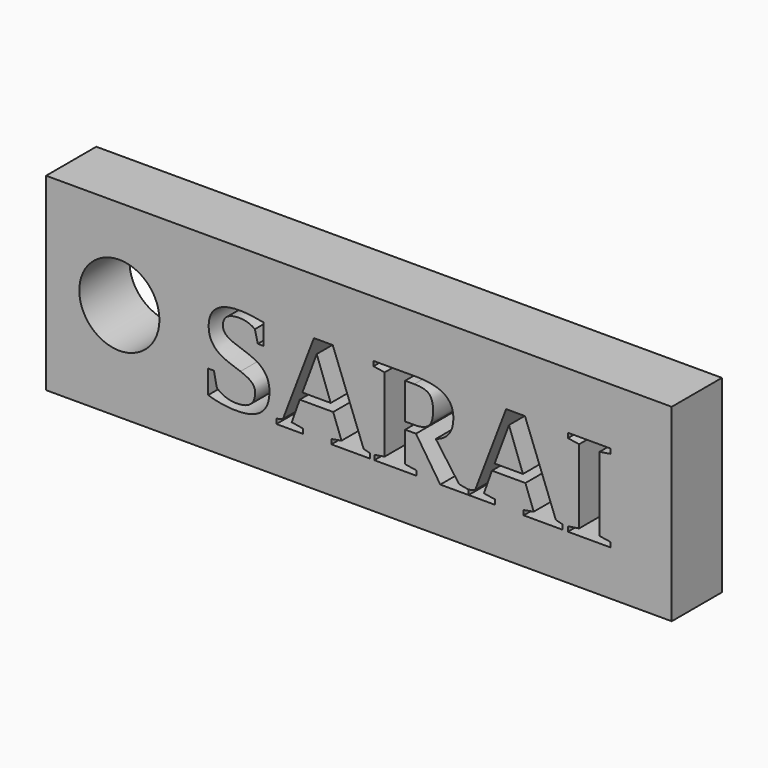
from build123d import *

# Parameters (mm, degrees)
F0_W         = 63.3234251291
F0_H         = 19.111122936
F1_DEPTH     = 6.35
F2_R         = 4.0540305713
F3_DEPTH     = 6.35
F4_TEXT_SIZE = 13.4696970539
F5_DEPTH     = 6.35


# Not quite as in the source:
# - Text() gives the source's letters only with a copy of the font that has no kerning and outlines rounded to 1/6400 em; it was checked with that copy


with BuildPart() as f1:
    # F0 (on Front) → F1 (new body)
    with BuildSketch(Plane.XZ):
        with Locations((1.8540648744, -0.4278607666)):
            Rectangle(F0_W, F0_H)
    extrude(amount=F1_DEPTH)

    # F2 (on face) → F3 (cut)
    with BuildSketch(Plane.XZ.offset(6.35)):
        with Locations((-22.3913900554, 0)):
            Circle(F2_R)
    extrude(amount=-F3_DEPTH, mode=Mode.SUBTRACT)

    # F4 (on face) → F5 (cut)
    with BuildSketch(Plane.XZ.offset(6.35)):
        with Locations((-14.11941275, -5.4195724661)):
            Text('SARAI', F4_TEXT_SIZE, font='Tinos', font_style=FontStyle.BOLD, text_align=(TextAlign.LEFT, TextAlign.BOTTOM))
    extrude(amount=-F5_DEPTH, mode=Mode.SUBTRACT)


solid = f1.part
